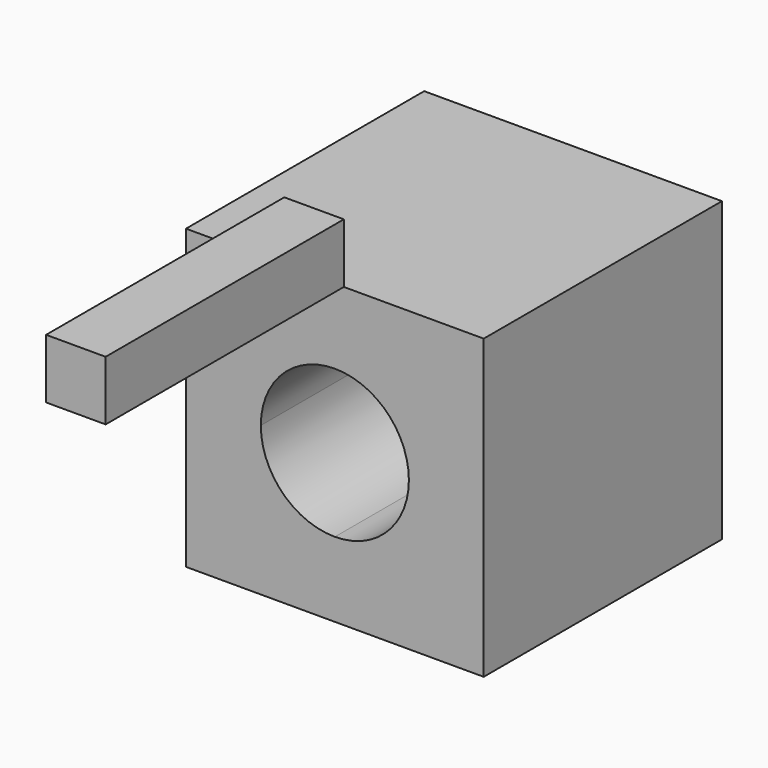
from build123d import *

# Parameters (mm, degrees)
F1_DEPTH = 50.8
F2_W     = 10.16
F2_H     = 10.16
F3_DEPTH = 50.8


# Not quite as in the source:
# - a feature names something its author has since deleted; it is built from what else it names


with BuildPart() as f1:
    # F0 (on Front) → F1 (new body)
    with BuildSketch(Plane.XZ):
        with BuildLine():
            Line((-41.48875705, 50.8), (-66.88875705, 50.8))
            Line((-66.88875705, 50.8), (-66.88875705, 25.4))
            Line((-66.88875705, 25.4), (-54.1182633227, 25.4))
            ThreePointArc((-54.1182633227, 25.4), (-50.4191665784, 34.3304095284), (-41.48875705, 38.0295062726))
            Line((-41.48875705, 38.0295062726), (-41.48875705, 50.8))
        make_face()
        with BuildLine():
            Line((-54.1182633227, 25.4), (-66.88875705, 25.4))
            Line((-66.88875705, 25.4), (-66.88875705, 0))
            Line((-66.88875705, 0), (-41.48875705, 0))
            Line((-41.48875705, 0), (-41.48875705, 12.7704937274))
            ThreePointArc((-41.48875705, 12.7704937274), (-50.4191665784, 16.4695904716), (-54.1182633227, 25.4))
        make_face()
        with BuildLine():
            Line((-16.08875705, 50.8), (-41.48875705, 50.8))
            Line((-41.48875705, 50.8), (-41.48875705, 38.0295062726))
            ThreePointArc((-41.48875705, 38.0295062726), (-32.5583475216, 34.3304095284), (-28.8592507774, 25.4))
            Line((-28.8592507774, 25.4), (-16.08875705, 25.4))
            Line((-16.08875705, 25.4), (-16.08875705, 50.8))
        make_face()
        with BuildLine():
            Line((-41.48875705, 12.7704937274), (-41.48875705, 0))
            Line((-41.48875705, 0), (-16.08875705, 0))
            Line((-16.08875705, 0), (-16.08875705, 25.4))
            Line((-16.08875705, 25.4), (-28.8592507774, 25.4))
            ThreePointArc((-28.8592507774, 25.4), (-32.5583475216, 16.4695904716), (-41.48875705, 12.7704937274))
        make_face()
    extrude(amount=F1_DEPTH)


with BuildPart() as f3:
    # F2 (on face) → F3 (new body)
    with BuildSketch(Plane.XZ.offset(50.8)):
        with Locations((-45.037239356, 55.88)):
            Rectangle(F2_W, F2_H)
    extrude(amount=F3_DEPTH)


solid = Compound([f1.part, f3.part])
